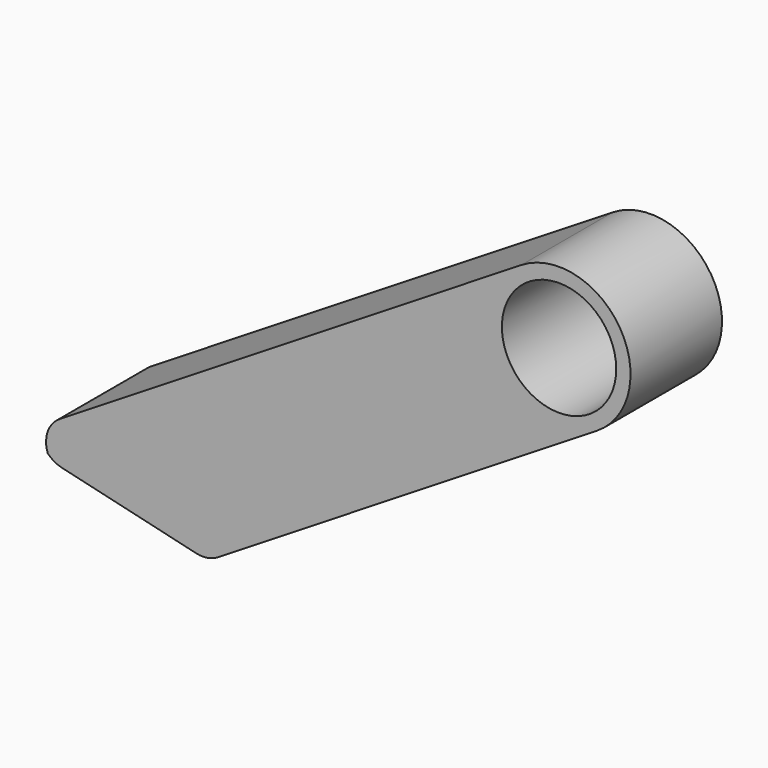
from build123d import *

# Parameters (mm, degrees)
F0_R        = 10
F1_DEPTH    = 20
F2_SIZE     = 20
F4_D        = 5
F4_DEPTH    = 10
F4_TIP      = 1.5021515476
F5_T1_DEPTH = 45
F5_T3_DEPTH = 30.3553390593


# Not quite as in the source:
# - a fillet or chamfer that OpenCascade refuses, or shapes differently, is made with other operations: its cross-section is extruded or revolved along the edge and cut away or added
# - a feature names something its author has since deleted; it is built from what else it names


with BuildPart() as f1:
    # F0 (on Front) → F1 (new body)
    with BuildSketch(Plane.XZ):
        with BuildLine():
            ThreePointArc((11.2991514202, 6.738710196), (15.6399466463, 11.2840038059), (17.2200345341, 17.3672200162))
            ThreePointArc((17.2200345341, 17.3672200162), (10.8032507445, 28.2871321284), (-1.8590823519, 27.9957298365))
            ThreePointArc((-1.8590823519, 27.9957298365), (-5.9084752861, 10.7881031302), (11.2991514202, 6.738710196))
        make_face()
        with Locations((4.7200345341, 17.3672200162)):
            Circle(F0_R, mode=Mode.SUBTRACT)
        with BuildLine():
            ThreePointArc((11.2991514202, 6.738710196), (-5.9084752861, 10.7881031302), (-1.8590823519, 27.9957298365))
            Line((-1.8590823519, 27.9957298365), (-86.8871609141, -24.6372052518))
            Line((-86.8871609141, -24.6372052518), (-73.728927142, -45.8942248924))
            Line((-73.728927142, -45.8942248924), (11.2991514202, 6.738710196))
        make_face()
    extrude(amount=F1_DEPTH)

    # F2
    f2_edges = [f1.edges().sort_by_distance(p)[0] for p in [
        (-73.728927, -10, -45.894225),
    ]]
    chamfer(f2_edges, length=F2_SIZE)

    # F4
    with Locations(Plane(origin=(-10.8625851344, 0, -46.1598350898), x_dir=(0.9734103626, 0, -0.2290682563), z_dir=(-0.2290682563, 0, -0.9734103626))):
        with Locations((-61.2555916321, 10)):
            Hole(F4_D / 2, depth=F4_DEPTH)
            with Locations((0, 0, -(F4_DEPTH + F4_TIP / 2))):  # 118° drill point
                Cone(0, F4_D / 2, F4_TIP, mode=Mode.SUBTRACT)

    # F5: fillet of radius 5 on 3 edges, made by hand

    # F5_s2 → F5_t1 (cut)
    with BuildSketch(Plane.XZ.offset(-12.5)):
        with BuildLine():
            ThreePointArc((-84.2555141597, -28.8886091799), (-84.8711620445, -25.1116211441), (-82.635756986, -22.0055584974))
            Line((-82.635756986, -22.0055584974), (-86.8871609141, -24.6372052518))
            Line((-86.8871609141, -24.6372052518), (-84.2555141597, -28.8886091799))
        make_face()
    extrude(amount=F5_T1_DEPTH, mode=Mode.SUBTRACT)

    # F5_s4 → F5_t3 (cut)
    with BuildSketch(Plane.XZ.offset(-5.1776695297)):
        with BuildLine():
            ThreePointArc((-85.3455779368, -27.1276200138), (-84.0148714695, -28.5542396802), (-82.2395152901, -29.3630250722))
            Line((-82.2395152901, -29.3630250722), (-84.2555141597, -28.8886091799))
            Line((-84.2555141597, -28.8886091799), (-85.3455779368, -27.1276200138))
        make_face()
        with BuildLine():
            ThreePointArc((-58.7393102993, -34.8932219824), (-56.7895862922, -34.9610428559), (-54.9623222634, -34.2775740977))
            Line((-54.9623222634, -34.2775740977), (-56.7233114296, -35.3676378747))
            Line((-56.7233114296, -35.3676378747), (-58.7393102993, -34.8932219824))
        make_face()
    extrude(amount=F5_T3_DEPTH, mode=Mode.SUBTRACT)


solid = f1.part
